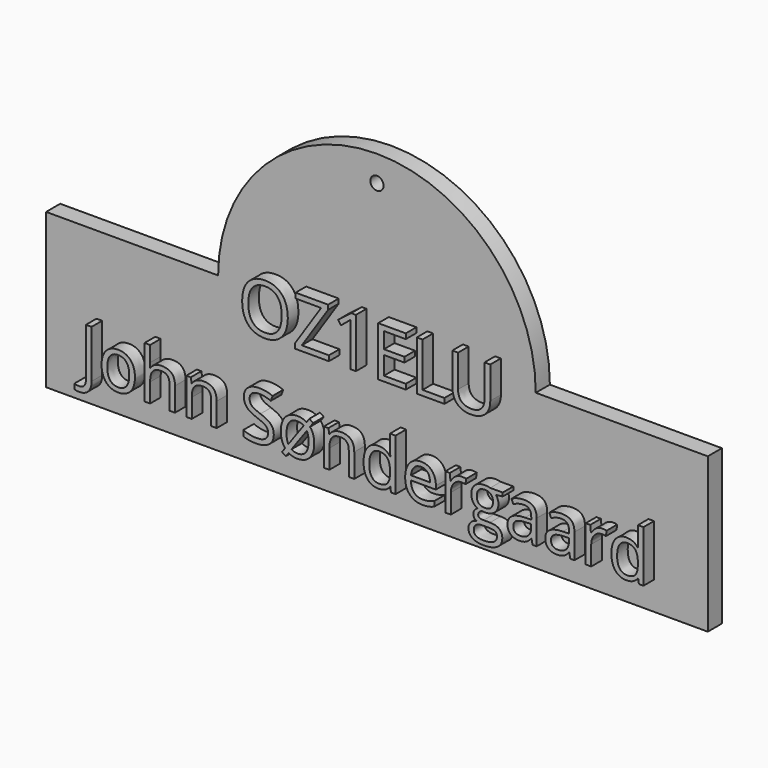
from build123d import *

# Parameters (mm, degrees)
F0_R           = 1.5
F1_DEPTH       = 4
F2_TEXT_SIZE   = 15.3928696971
F2_TEXT_SIZE_2 = 15.7405193352
F3_DEPTH       = 3


# Not quite as in the source:
# - Text() gives the source's letters only with a copy of the font that has no kerning and outlines rounded to 1/6400 em; it was checked with that copy


with BuildPart() as f1:
    # F0 (on Front) → F1 (new body)
    with BuildSketch(Plane.XZ):
        with BuildLine():
            Line((-75, 17.5), (-75, -17.5))
            Line((-75, -17.5), (75, -17.5))
            Line((75, -17.5), (75, 17.5))
            Line((75, 17.5), (35.999417305, 17.5))
            ThreePointArc((35.999417305, 17.5), (0, 53.499417305), (-35.999417305, 17.5))
            Line((-35.999417305, 17.5), (-75, 17.5))
        make_face()
        with Locations((0, 47.593344003)):
            Circle(F0_R, mode=Mode.SUBTRACT)
    extrude(amount=F1_DEPTH)

    # F2 (on face) → F3 (join)
    with BuildSketch(Plane.XZ.offset(4)):
        with Locations((-65, -11.0828661819)):
            Text('John Søndergaard', F2_TEXT_SIZE, font='Open Sans', text_align=(TextAlign.LEFT, TextAlign.BOTTOM))
        with Locations((-29.1076634894, 10.5418266374)):
            Text('OZ1ELU', F2_TEXT_SIZE_2, font='Open Sans', text_align=(TextAlign.LEFT, TextAlign.BOTTOM))
    extrude(amount=F3_DEPTH)


solid = f1.part
